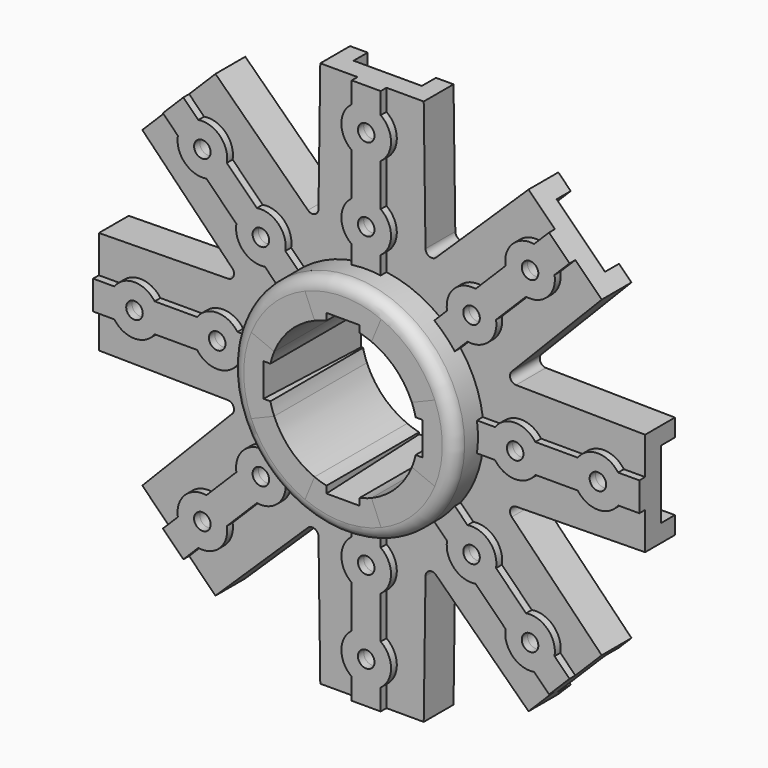
from build123d import *
from build123d import SkipClean  # not in build123d's __all__

# Parameters (mm, degrees)
F0_W             = 55.5625
F0_H             = 57.15
F0_W_2           = 57.15
F0_W_3           = 65.0875
F1_ANGLE_BACK    = 22.5
F1_ANGLE         = 45
F2_R             = 19.05
F0_H_2           = 247.65
F3_DEPTH         = 79.375
F4_R             = 12.7
F5_DEPTH         = 11.1125
F6_DEPTH         = 57.15
F7_DEPTH         = 122.2385
F8_W             = 104.775
F8_H             = 26.9875
F9_DEPTH         = 247.65
F10_COUNT        = 8
F11_R            = 9.525
F13_DEPTH        = 25.4
F13_COPIES_COUNT = 4


# Not quite as in the source:
# - a pattern or mirror of a feature is missing from the dataset's text; its kind, count and spacing are read off the source's solid


with BuildPart() as f1:
    # F0 (on Right) → F1 (revolve)
    with BuildSketch(Plane.YZ, mode=Mode.PRIVATE) as f1_sk:
        with Locations((-56.35625, 142.875)):
            Rectangle(F0_W, F0_H)
        with Locations((0, 142.875)):
            Rectangle(F0_W_2, F0_H)
        with Locations((61.11875, 142.875)):
            Rectangle(F0_W_3, F0_H)
    revolve(f1_sk.sketch.rotate(Axis((0, 4.7625, 0), (0, 1, 0)), -F1_ANGLE_BACK), axis=Axis((0, 4.7625, 0), (0, 1, 0)), revolution_arc=F1_ANGLE)

    # F2
    f2_edges = [f1.edges().sort_by_distance(p)[0] for p in [
        (0, -84.1375, 171.45),
        (0, 93.6625, 171.45),
    ]]
    fillet(f2_edges, radius=F2_R)

    # F0 (on Right) → F3 (join, symmetric)
    with BuildSketch(Plane.YZ):
        with Locations((0, 142.875)):
            Rectangle(F0_W_2, F0_H)
        with Locations((0, 295.275)):
            Rectangle(F0_W_2, F0_H_2)
    extrude(amount=F3_DEPTH, both=True)

    # F4 (on face) → F5 (join)
    with BuildSketch(Plane.XZ.offset(28.575)):
        with BuildLine():
            Line((22.225, 419.1), (-22.225, 419.1))
            Line((-22.225, 419.1), (-22.225, 386.5460720448))
            ThreePointArc((-22.225, 386.5460720448), (0, 393.7), (22.225, 386.5460720448))
            Line((22.225, 386.5460720448), (22.225, 419.1))
        make_face()
        with BuildLine():
            Line((-22.225, 386.5460720448), (-22.225, 324.6539279552))
            ThreePointArc((-22.225, 324.6539279552), (0, 317.5), (22.225, 324.6539279552))
            Line((22.225, 324.6539279552), (22.225, 386.5460720448))
            ThreePointArc((22.225, 386.5460720448), (0, 393.7), (-22.225, 386.5460720448))
        make_face()
        with Locations((0, 355.6)):
            Circle(F4_R, mode=Mode.SUBTRACT)
        with BuildLine():
            Line((22.225, 386.5460720448), (22.225, 324.6539279552))
            ThreePointArc((22.225, 324.6539279552), (33.8997234502, 338.2098087992), (38.1, 355.6))
            ThreePointArc((38.1, 355.6), (33.8997234502, 372.9901912008), (22.225, 386.5460720448))
        make_face()
        with BuildLine():
            ThreePointArc((-22.225, 386.5460720448), (-38.1, 355.6), (-22.225, 324.6539279552))
            Line((-22.225, 324.6539279552), (-22.225, 386.5460720448))
        make_face()
        with BuildLine():
            Line((-22.225, 324.6539279552), (-22.225, 259.5460720448))
            ThreePointArc((-22.225, 259.5460720448), (0, 266.7), (22.225, 259.5460720448))
            Line((22.225, 259.5460720448), (22.225, 324.6539279552))
            ThreePointArc((22.225, 324.6539279552), (0, 317.5), (-22.225, 324.6539279552))
        make_face()
        with BuildLine():
            Line((-22.225, 259.5460720448), (-22.225, 197.6539279552))
            ThreePointArc((-22.225, 197.6539279552), (-11.674002242, 192.3325535548), (-7.2e-08, 190.5))
            ThreePointArc((-7.2e-08, 190.5), (11.6740021735, 192.3325535328), (22.225, 197.6539279552))
            Line((22.225, 197.6539279552), (22.225, 259.5460720448))
            ThreePointArc((22.225, 259.5460720448), (0, 266.7), (-22.225, 259.5460720448))
        make_face()
        with Locations((0, 228.6)):
            Circle(F4_R, mode=Mode.SUBTRACT)
        with BuildLine():
            ThreePointArc((-22.225, 259.5460720448), (-38.1, 228.6), (-22.225, 197.6539279552))
            Line((-22.225, 197.6539279552), (-22.225, 259.5460720448))
        make_face()
        with BuildLine():
            Line((22.225, 259.5460720448), (22.225, 197.6539279552))
            ThreePointArc((22.225, 197.6539279552), (33.8997234502, 211.2098087992), (38.1, 228.6))
            ThreePointArc((38.1, 228.6), (33.8997234502, 245.9901912008), (22.225, 259.5460720448))
        make_face()
        with BuildLine():
            Line((-22.225, 197.6539279552), (-22.225, 190.5))
            Line((-22.225, 190.5), (-7.2e-08, 190.5))
            ThreePointArc((-7.2e-08, 190.5), (-11.674002242, 192.3325535548), (-22.225, 197.6539279552))
        make_face()
        with BuildLine():
            Line((-22.225, 190.5), (-22.225, 170.0033878339))
            ThreePointArc((-22.225, 170.0033878339), (0, 171.45), (22.225, 170.0033878339))
            Line((22.225, 170.0033878339), (22.225, 190.5))
            Line((22.225, 190.5), (-7.2e-08, 190.5))
            Line((-7.2e-08, 190.5), (-22.225, 190.5))
        make_face()
        with BuildLine():
            Line((-7.2e-08, 190.5), (22.225, 190.5))
            Line((22.225, 190.5), (22.225, 197.6539279552))
            ThreePointArc((22.225, 197.6539279552), (11.6740021735, 192.3325535328), (-7.2e-08, 190.5))
        make_face()
    extrude(amount=F5_DEPTH)

    # F4 (on face) → F6 (join, through all)
    with BuildSketch(Plane.XZ.offset(28.575)):
        Polygon((-82.55, 190.5), (-79.375, 190.5), (-79.375, 419.1), align=None)
        Polygon((79.375, 419.1), (79.375, 190.5), (82.55, 190.5), align=None)
    extrude(amount=-F6_DEPTH)

    # F4 (on face) → F7 (cut, through all)
    with BuildSketch(Plane.XZ.offset(28.575)):
        with Locations((0, 355.6)):
            Circle(F4_R)
        with Locations((0, 228.6)):
            Circle(F4_R)
    extrude(amount=-F7_DEPTH, mode=Mode.SUBTRACT)

    # F8 (on face) → F9 (cut)
    with BuildSketch(Plane.XY.offset(419.1)):
        with Locations((0, 15.08125)):
            Rectangle(F8_W, F8_H)
    extrude(amount=-F9_DEPTH, mode=Mode.SUBTRACT)

    # F10: F1 ×8 about axis
    f10_axis = Axis((0, 4.7625, 0), (0, 1, 0))


with BuildPart() as f1_1:
    add(f1.part, clean=False)
    with SkipClean():  # cleaning this boolean's faces spoils the solid; the shape is the same uncleaned
        for i in range(1, F10_COUNT):
            add(f1.part.rotate(f10_axis, i * 360 / F10_COUNT), clean=False)

    # F11
    f11_edges = [f1_1.edges().sort_by_distance(p)[0] for p in [
        (-82.431833, 0, 199.008048),
        (82.431833, 0, 199.008048),
        (199.008048, 0, 82.431833),
        (199.008048, 0, -82.431833),
        (82.431833, 0, -199.008048),
        (-82.431833, 0, -199.008048),
        (-199.008048, 0, -82.431833),
        (-199.008048, 0, 82.431833),
    ]]
    fillet(f11_edges, radius=F11_R)

    # F12 (on Right) → F13 (cut, symmetric)
    with BuildSketch(Plane.YZ):
        Polygon((-84.1375, 0), (93.6625, 0), (93.6625, 114.3), (-84.1375, 122.0629156491), align=None)
    f13 = extrude(amount=F13_DEPTH, both=True, mode=Mode.SUBTRACT)

    # F13_copies: F13 ×4 about axis
    f13_copies_axis = Axis((0, 0, 0), (0, 1, 0))
    for i in range(1, F13_COPIES_COUNT):
        add(f13.rotate(f13_copies_axis, i * 360 / F13_COPIES_COUNT), clean=False, mode=Mode.SUBTRACT)


solid = f1_1.part
